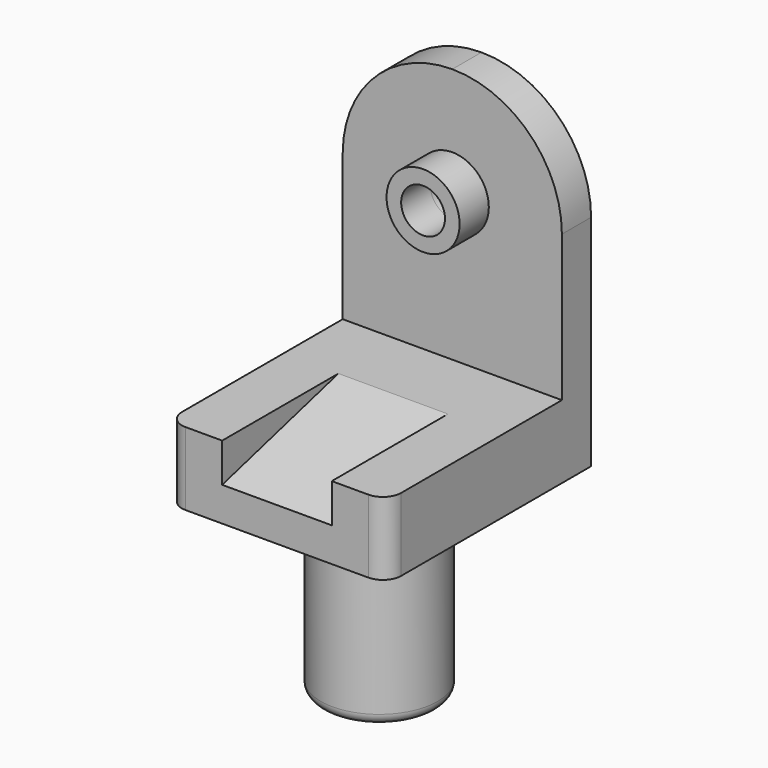
from build123d import *

# Parameters (mm, degrees)
F0_R      = 16
F1_DEPTH  = 50
F2_R      = 3
F3_R      = 16
F4_DEPTH  = 20
F7_DEPTH  = 15
F8_W      = 60
F8_H      = 10
F9_DEPTH  = 70
F10_R     = 29.99999
F11_R     = 10
F11_R_2   = 6
F12_DEPTH = 10
F13_DEPTH = 10.001


# Not quite as in the source:
# - a fillet or chamfer is up to 0.001 mm smaller than in the source, because OpenCascade refuses the exact size


with BuildPart() as f1:
    # F0 (on Top) → F1 (new body)
    with BuildSketch(Plane.XY):
        with Locations((-41.7741946876, 23.8037649542)):
            Circle(F0_R)
    extrude(amount=F1_DEPTH)

    # F2
    f2_edges = [f1.edges().sort_by_distance(p)[0] for p in [
        (-57.774195, 23.803765, 0),
    ]]
    fillet(f2_edges, radius=F2_R)

    # F3 (on face) → F4 (join)
    with BuildSketch(Plane.XY.offset(50)):
        with BuildLine():
            Line((-11.7741946876, 58.8037649542), (-41.7741946876, 58.8037649542))
            Line((-41.7741946876, 58.8037649542), (-71.7741946876, 58.8037649542))
            Line((-71.7741946876, 58.8037649542), (-71.7741946876, 23.8037649542))
            Line((-71.7741946876, 23.8037649542), (-71.7741946876, -6.1962350458))
            ThreePointArc((-71.7741946876, -6.1962350458), (-70.3097285935, -9.7317689517), (-66.7741946876, -11.1962350458))
            Line((-66.7741946876, -11.1962350458), (-56.7741946876, -11.1962350458))
            Line((-56.7741946876, -11.1962350458), (-41.7741946876, -11.1962350458))
            Line((-41.7741946876, -11.1962350458), (-26.7741946876, -11.1962350458))
            Line((-26.7741946876, -11.1962350458), (-16.7741946876, -11.1962350458))
            ThreePointArc((-16.7741946876, -11.1962350458), (-13.2386607817, -9.7317689517), (-11.7741946876, -6.1962350458))
            Line((-11.7741946876, -6.1962350458), (-11.7741946876, 58.8037649542))
        make_face()
        with Locations((-41.7741946876, 23.8037649542)):
            Circle(F3_R, mode=Mode.SUBTRACT)
        with Locations((-41.7741946876, 23.8037649542)):
            Circle(F3_R)
    extrude(amount=F4_DEPTH)

    # F6 (on offset) → F7 (cut, symmetric)
    with BuildSketch(Plane(origin=(-41.7741946876, 0, 0), x_dir=(0, -1, 0), z_dir=(-1, 0, 0))):
        Polygon((11.2580982968, 59.3282932557), (11.2580982968, 70.0462609529), (-28.7419017032, 70.0462609529), align=None)
    extrude(amount=F7_DEPTH, both=True, mode=Mode.SUBTRACT)

    # F8 (on face) → F9 (join)
    with BuildSketch(Plane.XY.offset(70)):
        with Locations((-41.7741946876, 53.8037649542)):
            Rectangle(F8_W, F8_H)
    extrude(amount=F9_DEPTH)

    # F10 (radius 30 in the source; OpenCascade refuses exactly that, so slightly less here)
    f10_edges = [f1.edges().sort_by_distance(p)[0] for p in [
        (-71.774195, 53.803765, 140),
        (-11.774195, 53.803765, 140),
    ]]
    fillet(f10_edges, radius=F10_R)

    # F11 (on face) → F12 (join)
    with BuildSketch(Plane.XZ.offset(-48.8037649542)):
        with Locations((-41.7741946876, 110)):
            Circle(F11_R)
        with Locations((-41.7741946876, 110)):
            Circle(F11_R_2, mode=Mode.SUBTRACT)
    extrude(amount=F12_DEPTH)

    # F13 (cut, through all): a face of the model
    f13_faces = [f1.faces().sort_by_distance(p)[0] for p in [
        (-41.7741946876, 48.8037649542, 110),
    ]]
    extrude(f13_faces, amount=-F13_DEPTH, mode=Mode.SUBTRACT)


solid = f1.part
